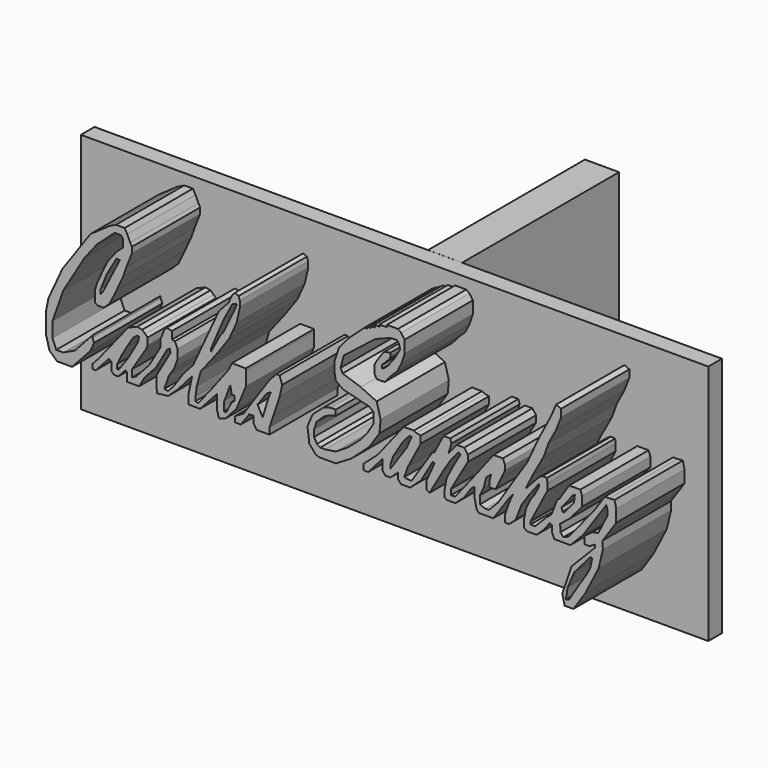
from build123d import *

# Parameters (mm, degrees)
F1_DEPTH = 25.4
F2_W     = 186.785928905
F2_H     = 71.9514414668
F3_DEPTH = 5.08
F5_DEPTH = 10.16


# Not quite as in the source:
# - a feature names something its author has since deleted; it is built from what else it names


with BuildPart() as f1:
    # F0 (on Front) → F1 (new body)
    with BuildSketch(Plane.XZ):
        Polygon((-65.4386132956, 33.3988890052), (-63.7945532799, 37.5722795725), (-63.7945532799, 39.279576391), (-64.3004179001, 40.2280725539), (-65.1856809855, 42.1250686049), (-65.9444779158, 43.5162000358), (-68.5370415449, 43.5162000358), (-70.5605000257, 42.5044670701), (-76.1250257492, 38.6312967342), (-84.5128575349, 26.7218568602), (-88.6451974511, 17.7170541137), (-89.3407613039, 14.2392273992), (-89.3407613039, 7.8526744619), (-88.3308967085, 4.101682537), (-86.052633822, 2.0227681249), (-81.6055082471, 2.0227681249), (-78.0506159677, 5.9185413701), (-76.1250257492, 8.028777705), (-75.0500634313, 10.4452362284), (-75.5283949538, 11.646666564), (-75.5283949538, 12.3005086801), (-76.1250257492, 11.646666564), (-80.7410478592, 6.5880110487), (-84.2188745737, 4.9439477734), (-86.3055661321, 4.9439477734), (-87.4437689781, 7.6629752293), (-87.4437689781, 12.0892990381), (-84.2188745737, 21.1948808283), (-77.9205225481, 31.7743477344), (-75.3309215045, 35.086631687), (-74.2280259728, 36.4973135293), (-68.9493492246, 41.2758216262), (-66.9651329517, 41.2758216262), (-66.4563626051, 40.4617860913), (-66.4563626051, 38.1977446377), (-68.3473423123, 36.4973135293), (-71.066364646, 33.01949054), (-74.0383267403, 26.7594028264), (-74.7338905931, 24.6094726026), (-74.7338905931, 21.1316477507), (-74.0383267403, 20.5625481904), (-72.204567492, 20.5625481904), (-70.3075677156, 22.3963111639), (-68.3473423123, 26.4432355762), (-66.3871094584, 30.6798610836), align=None)
        Polygon((-68.3473423123, 34.7267836332), (-67.3988461494, 34.6003174782), (-72.4574998021, 24.6094726026), (-73.0911253082, 23.9150883288), (-73.0911253082, 25.1153372228), (-71.3227370159, 29.6043309018), align=None, mode=Mode.SUBTRACT)
    extrude(amount=F1_DEPTH)


with BuildPart() as f1b:
    # F0 (on Front) → F1, piece 2 (new body)
    with BuildSketch(Plane.XZ):
        Polygon((-30.5617135018, 6.3387812115), (-33.0278091133, 4.9476511776), (-33.0278091133, 3.2403548248), (-31.3837453723, 3.2403548248), (-28.8471251119, 6.7683305423), (-27.6529863477, 6.7683305423), (-27.6529863477, 4.9476511776), (-26.6412552446, 3.3668212127), (-22.8472650051, 3.3668212127), (-22.8472650051, 5.2638174966), (-21.6458328068, 8.8048763573), (-19.7488367558, 14.4326305017), (-19.0532710403, 17.6575239748), (-19.8120698333, 19.8756745913), (-20.8232030269, 19.8756745913), (-22.8472650051, 17.6575239748), (-26.8309544772, 11.8400696665), align=None)
        Polygon((-22.8472650051, 13.8002987951), (-24.8707253486, 7.2240461595), (-26.3777443343, 10.135094718), (-23.6060619354, 13.989998959), (-22.1990532922, 14.7018429555), align=None, mode=Mode.SUBTRACT)
    extrude(amount=F1_DEPTH)


with BuildPart() as f1c:
    # F0 (on Front) → F1, piece 3 (new body)
    with BuildSketch(Plane.XZ):
        Polygon((-73.7742282088, 6.6766220952), (-75.5283949538, 4.7542471439), (-75.5283949538, 4.2483815923), (-75.5283949538, 3.4263499547), (-74.5441913605, 3.4263499547), (-70.6534928755, 7.690130084), (-69.9113289495, 7.2633184893), (-69.9113289495, 4.7542471439), (-69.0747495214, 3.990868589), (-67.8414776921, 3.990868589), (-65.7261914464, 6.3089910283), (-65.2074660032, 5.8356541689), (-65.2074660032, 3.4263499547), (-61.6446211934, 3.4263499547), (-59.986841031, 6.3089910283), (-56.5836195384, 10.0385496749), (-53.2882678202, 15.7686919642), (-52.5390431285, 16.3259226829), (-52.2861070931, 15.250957571), (-56.4536216041, 8.0042497282), (-56.4536216041, 4.7542471439), (-56.2697984278, 3.2998835668), (-52.9711393333, 3.7168150699), (-50.1361787319, 6.3089910283), (-45.8363220096, 11.2672662362), (-46.9112880528, 6.3089910283), (-46.9112880528, 3.4263499547), (-43.4966944158, 3.4263499547), (-41.1538538285, 5.9938470715), (-38.4564168185, 8.9499430959), (-38.4564168185, 4.7542471439), (-37.8689393401, 2.7307847049), (-36.0272358169, 3.2654916117), (-32.6621944215, 6.9532090464), (-29.8383217305, 13.7333609164), (-29.8383217305, 17.9067514837), (-29.8661477864, 18.4596965993), (-31.95284307, 18.4596965993), (-34.0201964633, 18.4596965993), (-34.8768906481, 16.5825616568), (-40.2363911271, 9.5004430041), (-44.0913048408, 4.6635263261), (-44.8524169624, 5.0108856522), (-44.8524169624, 6.275549531), (-44.4730184972, 9.0578105301), (-43.2715862989, 13.3576681837), (-38.7187935412, 19.1751215607), (-34.8768906481, 24.5536185025), (-33.9484848082, 26.5878835575), (-32.6581449885, 29.4151958078), (-31.6088534892, 33.9679867029), (-31.6720865667, 35.6752835214), (-32.0248657335, 36.7211668581), (-33.1165048342, 37.2193733792), (-33.9484848082, 36.3076142967), (-34.9908635544, 34.0236189075), (-37.8689430654, 30.8695584536), (-45.5560506462, 14.2198124948), (-48.3656488359, 11.1408000812), (-51.2116778089, 6.9789612562), (-53.0544459368, 4.9594888768), (-54.1442914778, 5.1774575181), (-53.7029706198, 6.442579911), (-52.7919754386, 9.0541047975), (-51.1258493176, 11.646666564), (-50.1994118094, 14.3024595454), (-50.1994118094, 16.9582553208), (-50.9920103839, 18.6862602302), (-51.8369585892, 18.8552495092), (-51.8369585892, 21.1009970089), (-53.4219470776, 21.4179940275), (-54.198688991, 20.5667698196), (-55.3213022649, 17.7170541137), (-55.3213022649, 15.693590045), (-58.5734635655, 10.0385496749), (-62.5298842788, 5.7027451694), (-63.7945532799, 5.0071799196), (-63.7945532799, 7.1571087465), (-59.5239674411, 13.9250130678), (-59.0763564669, 15.0612583384), (-59.0763564669, 17.0580966179), (-59.7985018318, 17.7170541137), (-60.7180135087, 18.5561083285), (-62.2137226164, 18.8552495092), (-64.9327486753, 17.7170541137), align=None)
        Polygon((-64.9857744575, 9.6138678491), (-67.83490628, 5.6454348378), (-68.1910514832, 5.7980669662), (-68.1910514832, 7.12087797), (-66.8173581362, 9.919132106), (-65.3419196606, 12.5138768926), (-63.3577033877, 15.6682729721), (-62.1775495363, 16.5555547071), (-61.6278722882, 16.43143408), (-61.9840137661, 14.8542355746), align=None, mode=Mode.SUBTRACT)
        Polygon((-36.4213697612, 6.4870067872), (-36.2954549491, 7.8001208603), (-34.4966687262, 12.5489160419), (-34.0649597347, 10.2104935795), (-33.2734920084, 10.2104935795), (-33.1835523248, 9.6528707072), (-33.1835523248, 9.0232957155), (-33.5253216326, 8.4656719118), (-34.0289846063, 8.3757322282), (-34.298799932, 7.7101816423), (-34.568618983, 7.2065214626), (-34.8744131625, 6.6309100948), (-35.2701470256, 6.0373106971), (-35.2701470256, 5.5156624876), (-35.8457565308, 5.5336505175), (-35.8457565308, 4.9940147437), (-36.4393554628, 4.9940147437), align=None, mode=Mode.SUBTRACT)
        Polygon((-32.0424485574, 15.5890771529), (-31.0063022562, 16.9582553208), (-30.6661876739, 16.700868463), (-30.6661876739, 14.4125586376), (-31.8000800908, 12.5087341294), (-31.8000800908, 11.3536044955), (-32.8268632293, 11.3536044955), (-32.8696444631, 12.4659510329), (-32.8696444631, 13.7922111899), align=None, mode=Mode.SUBTRACT)
        Polygon((-32.6581449885, 34.4775542617), (-32.6581449885, 33.9679867029), (-33.9738164914, 31.085169246), (-36.5056321025, 25.8146058768), (-37.4541319907, 24.6764086187), (-40.1731580496, 19.5545200258), (-40.1731580496, 20.4397849739), (-36.5056321025, 29.0395002812), (-33.8892762859, 33.9679867029), align=None, mode=Mode.SUBTRACT)
        Polygon((-30.6661876739, 16.700868463), (-31.0063022562, 16.9582553208), (-32.0424485574, 15.5890771529), (-32.8696444631, 13.7922111899), (-32.8696444631, 12.4659510329), (-32.8268632293, 11.3536044955), (-31.8000800908, 11.3536044955), (-31.8000800908, 12.5087341294), (-30.6661876739, 14.4125586376), align=None)
    extrude(amount=F1_DEPTH)


with BuildPart() as f1d:
    # F0 (on Front) → F1, piece 4 (new body)
    with BuildSketch(Plane.XZ):
        Polygon((-10.9813613817, 4.8844176345), (-9.1256611049, 2.6712561958), (-7.9306939194, 2.2684582103), (-3.0552726239, 2.2684582103), (1.4342841459, 4.9476511776), (6.7458730191, 9.690140374), (9.9040192077, 14.3470675708), (10.2443126962, 18.0850736797), (9.0855006129, 22.4632453173), (4.3430095538, 24.676406756), (-1.056341731, 26.4964130682), (-1.6636506189, 27.7625415474), (-0.7010490519, 31.3167614803), (8.6973570287, 38.6991612613), (13.1583465263, 40.4259972274), (15.137010254, 40.4979474843), (15.7485976815, 39.6345295012), (16.0723794252, 38.3394025266), (15.4248159379, 37.2601300478), (14.7053021938, 35.9290316701), (13.9498123899, 34.8137840629), (12.3668797314, 32.8351184726), (11.4674875513, 32.0436544716), (10.6760216877, 31.539991498), (10.6040704995, 32.4753597379), (12.9065159708, 34.8137840629), (13.2338090921, 35.7847535166), (13.2302977145, 36.5765951574), (11.3595603034, 36.2168364227), (10.9278513119, 35.7491523027), (10.2802887559, 34.8137840629), (9.2010172084, 33.2668274641), (8.481502533, 32.0796296), (8.4455264732, 31.0003571212), (8.3735752851, 29.5613277704), (9.0855006129, 28.3021777868), (11.4315114915, 28.3021777868), (13.1393406276, 30.311388187), (15.137010254, 32.2595052421), (16.3961611688, 34.6698798239), (17.4246560622, 37.7210809035), (17.4246560622, 41.361361742), (16.3961593062, 42.8363643587), (15.4248150066, 43.5199029744), (12.1150491759, 43.5199029744), (12.1150491759, 42.9083183408), (9.9040192077, 42.9083183408), (10.1004084572, 42.3327051103), (8.3735752851, 42.3327051103), (8.5894288495, 41.6491664946), (7.3302784003, 41.6491664946), (7.3302784003, 41.1455072463), (6.2869829126, 41.1455072463), (6.2869829126, 40.6058728695), (5.4595409892, 40.6058728695), (4.4162450358, 39.6705009043), (0.5855057039, 36.145206517), (-2.0791381479, 33.0103319404), (-3.534415424, 28.6930099738), (-3.534415424, 26.320470497), (-3.0552740209, 23.9176098257), (-0.9053455433, 22.3367791623), (2.0666148048, 21.6412153095), (5.1018083468, 20.819183439), (6.7458720878, 20.4397849739), (8.0737695098, 19.4912869483), (8.2002356648, 17.6575239748), (8.2002356648, 16.392858699), (6.366473157, 13.3576663211), (4.2165433988, 10.8283376321), (0.6754847127, 7.7299117111), (-3.0552740209, 5.390283186), (-6.2801670283, 4.8844176345), (-7.7345306054, 4.8844176345), (-8.7148919702, 5.5295475759), (-9.5423329622, 7.076503709), (-9.5423329622, 9.0551683679), (-8.7508670986, 11.3576147705), (-6.5563484095, 13.4442057461), (-4.9014654942, 14.2716476694), (-3.1026795041, 14.7033557296), (-3.1026795041, 16.3582395762), (-4.5057325624, 16.3582395762), (-6.6642756574, 15.7826282084), (-9.9740419537, 12.8685943782), (-11.5209976211, 9.3069979921), align=None)
    extrude(amount=F1_DEPTH)


with BuildPart() as f1e:
    # F0 (on Front) → F1, piece 5 (new body)
    with BuildSketch(Plane.XZ):
        Polygon((9.4981548348, 8.6968088431), (5.2282758988, 4.8844176345), (5.2282758988, 3.1771215145), (6.5561723895, 3.1138886698), (10.7927974313, 7.9196114093), (10.7927974313, 4.8844176345), (11.7442116684, 3.8188334938), (13.1956581026, 3.8726869971), (15.4210715892, 5.8596629603), (15.4210715892, 4.1256193072), (16.3244023499, 3.1138886698), (19.0131124109, 3.1138886698), (22.2450513425, 5.9995479013), (25.8422978222, 12.1562359855), (26.3216467568, 11.8761606846), (25.2099651843, 9.3739749864), (23.9453017712, 6.591714453), (23.9453017712, 4.0623862296), (24.8305667192, 3.6197542213), (29.1304234415, 11.1445048824), (31.0906525701, 14.1796981916), (33.4302820265, 17.0884244144), (34.0387347215, 16.5990164265), (31.9126844406, 12.9782669246), (29.8892222345, 9.1210417449), (29.3201245368, 5.8961492032), (29.3201245368, 3.9359200746), (29.7627560794, 3.4300542902), (32.5450152159, 3.4300542902), (34.9966159832, 5.6189831457), (37.4772064388, 9.1210417449), (38.2360033691, 9.5004411414), (38.2360033691, 6.591714453), (38.8683378696, 3.809453221), (39.4893775338, 3.1138886698), (43.8005253673, 3.1138886698), (48.2900813222, 9.6269072965), (49.6812127531, 11.334204115), (48.4165474772, 8.4887100384), (47.2783520818, 5.2005834877), (47.2783520818, 3.1138886698), (48.4797805548, 3.1138886698), (50.4627733586, 4.8844176345), (52.2737763822, 9.5004411414), (54.739870131, 13.104734011), (57.3956631124, 16.5825597942), (57.3956631124, 15.7605279237), (55.941298604, 13.0415000021), (54.8133219418, 11.5643870095), (53.5384379327, 8.8681094348), (52.969340235, 5.8961492032), (52.969340235, 3.6197542213), (53.812472922, 2.9759077459), (56.7000992596, 2.9759077459), (58.7867945433, 4.947650712), (60.6606568163, 7.4015191321), (61.2844727551, 6.9251508218), (61.2528882921, 5.2005830221), (61.9484558702, 3.5565195139), (64.098380506, 3.5565195139), (66.7541772127, 3.5565195139), (70.4849362373, 7.4015191321), (77.4405896664, 17.5310559571), (77.7694038959, 16.4560917765), (77.7694038959, 14.8373209093), (75.0377252698, 9.3739731237), (73.3936652541, 9.1210398823), (70.92756778, 7.3505113833), (70.92756778, 5.1373485476), (72.5084021688, 5.1373485476), (74.1524621844, 6.1490801163), (74.1524621844, 5.3270487115), (67.0703426003, -1.9447690574), (64.3513128161, -9.9121518433), (65.0468841195, -12.8917823924), (67.6477684423, -12.8917823924), (68.7050458017, -11.3187569411), (71.1805000901, -7.6357568614), (75.1641914248, 0.2051601914), (76.4099999371, 5.4547837963), (76.3414755084, 7.8531438459), (77.8199881315, 10.0063057616), (80.4125443101, 13.8635309413), (80.4125443101, 17.4678228796), (79.9066796899, 19.6809843183), (78.3258527517, 19.5776981958), (77.0219003764, 19.5776981958), (73.8362967968, 14.9384951219), (66.31154567, 5.6432154961), (64.6674782038, 4.9476502463), (63.7822151184, 5.9593813494), (63.7189820409, 8.1725437194), (66.5644779801, 10.4489382356), (70.2320039272, 14.7487958893), (70.2320039272, 17.5942890346), (69.726139307, 19.0614008174), (67.9556056857, 19.0614008174), (66.3802096557, 19.0614008174), (63.5292828083, 14.6855628118), (62.8337189555, 14.1796972603), (61.126422137, 9.7533734515), (59.5455914736, 8.4254760295), (56.2574639916, 5.0741164014), (54.8663362861, 5.0741164014), (54.8663362861, 5.8961478062), (59.9249899387, 15.5708277598), (59.9249899387, 17.5942908973), (59.7352907062, 18.8589524478), (58.5338622332, 18.9854204655), (57.3956593871, 18.28985475), (53.4119680524, 13.9899980277), (55.5619001389, 18.28985475), (58.8500238955, 24.2337752134), (60.3043884039, 28.2807014883), (62.5175535679, 32.390858978), (63.9967899702, 36.1848510802), (63.9967899702, 38.4090629943), (62.5175535679, 39.0303432941), (61.1896552145, 35.8686856925), (57.1427308023, 28.0910022557), (53.9810732007, 21.1985837668), (48.5430136323, 12.8518007696), (45.2548898757, 7.7299121767), (42.4726307392, 4.8844181001), (41.397664696, 4.8844181001), (39.8168340325, 5.4535167292), (39.8168340325, 7.8563783318), (40.9550331533, 10.1960068569), (41.7138300836, 13.1679670885), (43.168194592, 14.4326305017), (42.6068004692, 12.4910181829), (42.7255630493, 10.8283385634), (44.4960929453, 10.9548047185), (46.140152961, 14.3693974242), (47.2783520818, 16.7722590268), (47.2783520818, 18.3530896902), (46.6460213065, 19.7442192584), (43.8637584448, 19.7442192584), (38.6154055595, 12.9150338471), (35.137578845, 8.4887100384), (32.4185490608, 5.0741173327), (31.2171205878, 5.0741173327), (31.2171205878, 6.718180608), (34.0626128018, 11.7136035115), (36.212541163, 15.3811285272), (36.212541163, 17.3413585871), (35.137578845, 18.8161514659), (32.9161078838, 18.8161514659), (30.4583217949, 15.7605279237), (31.3435867429, 18.6692550778), (30.9641864151, 19.8826261284), (28.9811952967, 19.8826261284), (26.2216962874, 14.6223306656), (25.7790647447, 14.6223306656), (19.4557439536, 5.0108842552), (17.8018438122, 5.152375006), (17.3058155924, 5.3270501085), (18.3765314441, 8.3675823322), (20.6601229094, 12.7206789571), (22.1884544935, 15.634061303), (22.1884544935, 17.7612005659), (20.910108462, 18.0369224399), (20.151309669, 18.4163227677), (17.1161163598, 18.4163227677), align=None)
        Polygon((71.338839829, -2.9959874228), (69.201990962, -6.2521379441), (66.4037391543, -10.7802217826), (65.3861910105, -11.1363632604), (65.945841372, -7.8293355182), (67.9300576448, -3.1486195512), (72.8142857552, 2.4478889536), (73.2254350737, 2.0890675461), (72.661653161, -0.6047519855), align=None, mode=Mode.SUBTRACT)
        Polygon((17.938144505, 13.1047321483), (13.1956543773, 6.149080582), (13.2062856565, 7.2829847004), (14.0176862478, 9.6901394427), (16.7999472469, 14.3061634153), (18.8866425306, 16.7090240866), (19.5189751685, 16.519324854), align=None, mode=Mode.SUBTRACT)
        Polygon((67.8035172513, 14.9356991646), (64.8987963796, 11.5301646292), (64.4147619605, 11.5301646292), (64.1160333485, 12.6320153667), (66.1693736911, 15.0393797085), (67.137427628, 16.4914689958), (68.1054890156, 17.2175131738), align=None, mode=Mode.SUBTRACT)
    extrude(amount=F1_DEPTH)


with BuildPart() as f3:
    # F2 (on Front) → F3 (new body)
    with BuildSketch(Plane.XZ):
        with Locations((-5.9031359851, 10.7927173376)):
            Rectangle(F2_W, F2_H)
    extrude(amount=-F3_DEPTH)

    # F4 (on Right) → F5 (join)
    with BuildSketch(Plane.YZ):
        Polygon((5.0366027281, -25.1830033958), (63.4611770511, -25.1830033958), (63.4611770511, 46.7805415392), (5.0703492016, 46.7805415392), align=None)
    extrude(amount=F5_DEPTH)


solid = Compound([f1.part, f1b.part, f1c.part, f1d.part, f1e.part, f3.part])
